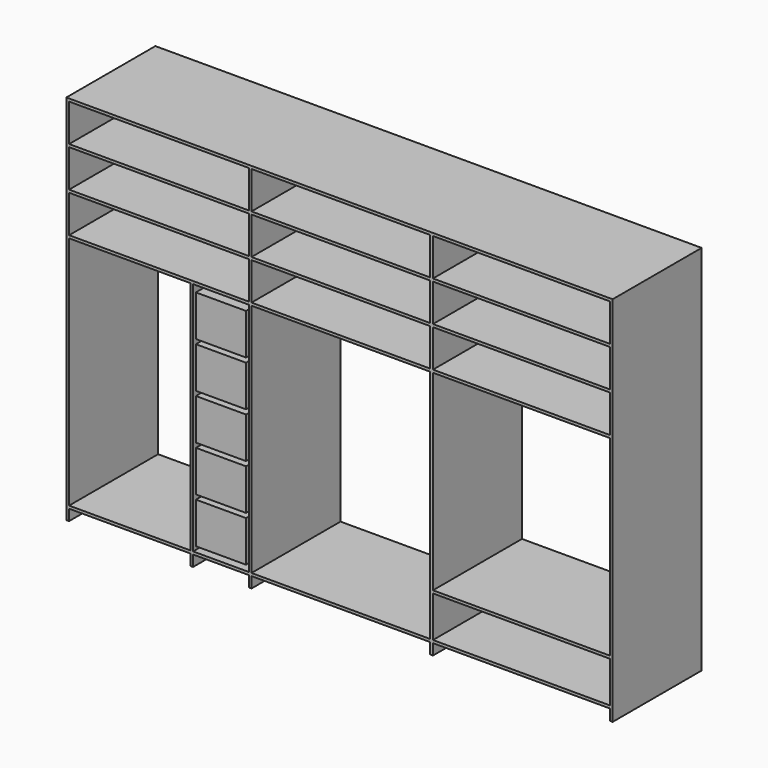
from build123d import *

# Parameters (mm, degrees)
F0_W     = 985
F0_H     = 15
F0_W_2   = 665
F0_W_3   = 305
F0_W_4   = 980
F0_W_5   = 970
F1_DEPTH = 610
F3_DEPTH = 2965
F0_W_6   = 275
F0_H_2   = 225
F4_DEPTH = 610


with BuildPart() as f1:
    # F0 (on Front) → F1 (new body)
    with BuildSketch(Plane.XZ):
        Polygon((1268.9268333363, 1797.1661111622), (1253.9268333363, 1797.1661111622), (1253.9268333363, 1782.1661111622), (1253.9268333363, 1577.1661111622), (1253.9268333363, 1562.1661111622), (1253.9268333363, 1357.1661111622), (1253.9268333363, 1342.1661111622), (1253.9268333363, 1137.1661111622), (1253.9268333363, 1122.1661111622), (1253.9268333363, -167.8338888378), (1253.9268333363, -182.8338888378), (1253.9268333363, -242.8338888378), (1268.9268333363, -242.8338888378), (1268.9268333363, -182.8338888378), (1268.9268333363, -167.8338888378), (1268.9268333363, 1122.1661111622), (1268.9268333363, 1137.1661111622), (1268.9268333363, 1342.1661111622), (1268.9268333363, 1357.1661111622), (1268.9268333363, 1562.1661111622), (1268.9268333363, 1577.1661111622), (1268.9268333363, 1782.1661111622), align=None)
        Polygon((268.9268333363, 1797.1661111622), (253.9268333363, 1797.1661111622), (253.9268333363, -242.8338888378), (268.9268333363, -242.8338888378), (268.9268333363, -182.8338888378), (268.9268333363, -167.8338888378), (268.9268333363, 1122.1661111622), (268.9268333363, 1137.1661111622), (268.9268333363, 1342.1661111622), (268.9268333363, 1357.1661111622), (268.9268333363, 1562.1661111622), (268.9268333363, 1577.1661111622), (268.9268333363, 1782.1661111622), align=None)
        Polygon((933.9268333363, -167.8338888378), (933.9268333363, -182.8338888378), (933.9268333363, -242.8338888378), (948.9268333363, -242.8338888378), (948.9268333363, -182.8338888378), (948.9268333363, -167.8338888378), (948.9268333363, 1122.1661111622), (933.9268333363, 1122.1661111622), align=None)
        with Locations((761.4268333363, 1789.6661111622)):
            Rectangle(F0_W, F0_H)
        with Locations((761.4268333363, 1569.6661111622)):
            Rectangle(F0_W, F0_H)
        with Locations((761.4268333363, 1349.6661111622)):
            Rectangle(F0_W, F0_H)
        Polygon((268.9268333363, 1137.1661111622), (268.9268333363, 1122.1661111622), (933.9268333363, 1122.1661111622), (948.9268333363, 1122.1661111622), (1253.9268333363, 1122.1661111622), (1253.9268333363, 1137.1661111622), align=None)
        with Locations((601.4268333363, -175.3338888378)):
            Rectangle(F0_W_2, F0_H)
        with Locations((1101.4268333363, -175.3338888378)):
            Rectangle(F0_W_3, F0_H)
        with Locations((1758.9268333363, 1789.6661111622)):
            Rectangle(F0_W_4, F0_H)
        with Locations((2748.9268333363, 1789.6661111622)):
            Rectangle(F0_W_5, F0_H)
        with Locations((1758.9268333363, 1569.6661111622)):
            Rectangle(F0_W_4, F0_H)
        with Locations((2748.9268333363, 1569.6661111622)):
            Rectangle(F0_W_5, F0_H)
        with Locations((2748.9268333363, 1349.6661111622)):
            Rectangle(F0_W_5, F0_H)
        with Locations((1758.9268333363, 1349.6661111622)):
            Rectangle(F0_W_4, F0_H)
        with Locations((1758.9268333363, 1129.6661111622)):
            Rectangle(F0_W_4, F0_H)
        with Locations((2748.9268333363, 1129.6661111622)):
            Rectangle(F0_W_5, F0_H)
        Polygon((2263.9268333363, 1797.1661111622), (2248.9268333363, 1797.1661111622), (2248.9268333363, 1782.1661111622), (2248.9268333363, 1577.1661111622), (2248.9268333363, 1562.1661111622), (2248.9268333363, 1357.1661111622), (2248.9268333363, 1342.1661111622), (2248.9268333363, 1137.1661111622), (2248.9268333363, 1122.1661111622), (2248.9268333363, -167.8338888378), (2248.9268333363, -182.8338888378), (2248.9268333363, -242.8338888378), (2263.9268333363, -242.8338888378), (2263.9268333363, -182.8338888378), (2263.9268333363, -167.8338888378), (2263.9268333363, 57.1661111622), (2263.9268333363, 72.1661111622), (2263.9268333363, 1122.1661111622), (2263.9268333363, 1137.1661111622), (2263.9268333363, 1342.1661111622), (2263.9268333363, 1357.1661111622), (2263.9268333363, 1562.1661111622), (2263.9268333363, 1577.1661111622), (2263.9268333363, 1782.1661111622), align=None)
        Polygon((3248.9268333363, 1797.1661111622), (3233.9268333363, 1797.1661111622), (3233.9268333363, 1782.1661111622), (3233.9268333363, 1577.1661111622), (3233.9268333363, 1562.1661111622), (3233.9268333363, 1357.1661111622), (3233.9268333363, 1342.1661111622), (3233.9268333363, 1137.1661111622), (3233.9268333363, 1122.1661111622), (3233.9268333363, 72.1661111622), (3233.9268333363, 57.1661111622), (3233.9268333363, -167.8338888378), (3233.9268333363, -182.8338888378), (3233.9268333363, -242.8338888378), (3248.9268333363, -242.8338888378), align=None)
        with Locations((2748.9268333363, -175.3338888378)):
            Rectangle(F0_W_5, F0_H)
        with Locations((1758.9268333363, -175.3338888378)):
            Rectangle(F0_W_4, F0_H)
        with Locations((2748.9268333363, 64.6661111622)):
            Rectangle(F0_W_5, F0_H)
    extrude(amount=F1_DEPTH)


with BuildPart() as f3:
    # F2 (on face) → F3 (new body, through all)
    with BuildSketch(Plane.YZ.offset(268.9268333363)):
        with BuildLine():
            Line((-322.5, 1077.1661111622), (-322.5, 1057.1661111622))
            ThreePointArc((-322.5, 1057.1661111622), (-315, 1049.6661111622), (-307.5, 1057.1661111622))
            Line((-307.5, 1057.1661111622), (-307.5, 1077.1661111622))
            ThreePointArc((-307.5, 1077.1661111622), (-315, 1084.6661111622), (-322.5, 1077.1661111622))
        make_face()
    extrude(amount=F3_DEPTH)


with BuildPart() as f4:
    # F0 (on Front) → F4 (new body)
    with BuildSketch(Plane.XZ):
        with Locations((1101.4268333363, 974.6661111622)):
            Rectangle(F0_W_6, F0_H_2)
    extrude(amount=F4_DEPTH)


with BuildPart() as f4b:
    # F0 (on Front) → F4, piece 2 (new body)
    with BuildSketch(Plane.XZ):
        with Locations((1101.4268333363, 724.6661111622)):
            Rectangle(F0_W_6, F0_H_2)
    extrude(amount=F4_DEPTH)


with BuildPart() as f4c:
    # F0 (on Front) → F4, piece 3 (new body)
    with BuildSketch(Plane.XZ):
        with Locations((1101.4268333363, 474.6661111622)):
            Rectangle(F0_W_6, F0_H_2)
    extrude(amount=F4_DEPTH)


with BuildPart() as f4d:
    # F0 (on Front) → F4, piece 4 (new body)
    with BuildSketch(Plane.XZ):
        with Locations((1101.4268333363, 224.6661111622)):
            Rectangle(F0_W_6, F0_H_2)
    extrude(amount=F4_DEPTH)


with BuildPart() as f4e:
    # F0 (on Front) → F4, piece 5 (new body)
    with BuildSketch(Plane.XZ):
        with Locations((1101.4268333363, -25.3338888378)):
            Rectangle(F0_W_6, F0_H_2)
    extrude(amount=F4_DEPTH)


solid = Compound([f1.part, f3.part, f4.part, f4b.part, f4c.part, f4d.part, f4e.part])
